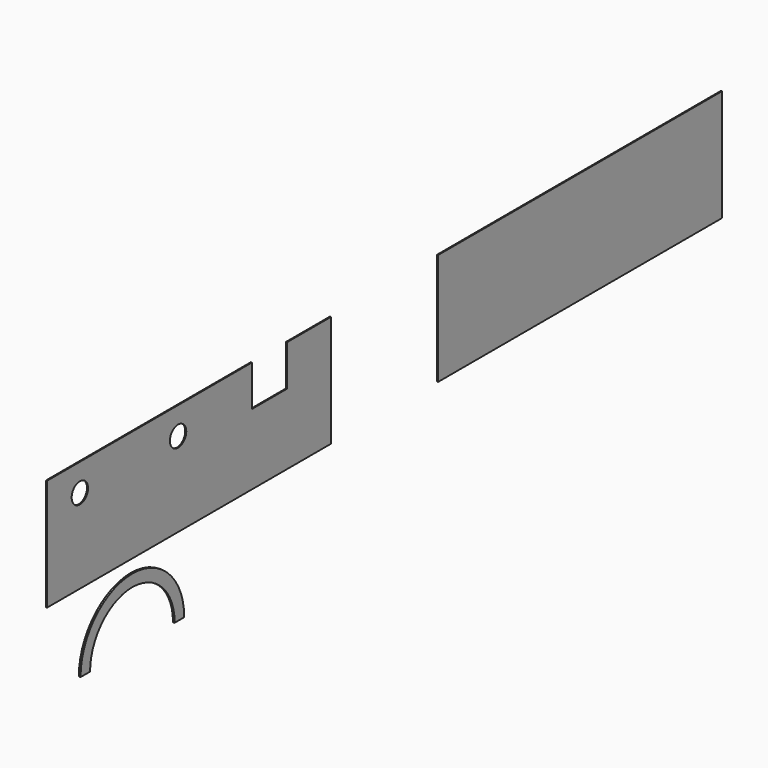
from build123d import *

# Parameters (mm, degrees)
F0_W     = 62
F0_H     = 32.75
F0_R     = 3
F1_DEPTH = 0.3
F0_W_2   = 104
F2_DEPTH = 0.5


# Not quite as in the source:
# - a feature names something its author has since deleted; it is built from what else it names


with BuildPart() as f1:
    # F0 (on Right) → F1 (new body)
    with BuildSketch(Plane.YZ):
        Polygon((-103.3088661638, 20.0492352203), (-61.3088661638, 20.0492352203), (-61.3088661638, 52.7992352203), (-77.3088661638, 52.7992352203), (-77.3088661638, 40.7992352203), (-90.3088661638, 40.7992352203), (-90.3088661638, 52.7992352203), (-103.3088661638, 52.7992352203), align=None)
        with Locations((-134.3088661638, 36.4242352203)):
            Rectangle(F0_W, F0_H)
        with Locations((-153.3088661638, 44.7992352203)):
            Circle(F0_R, mode=Mode.SUBTRACT)
        with Locations((-117.3088661638, 44.7992352203)):
            Circle(F0_R, mode=Mode.SUBTRACT)
    extrude(amount=F1_DEPTH)


with BuildPart() as f1b:
    # F0 (on Right) → F1, piece 2 (new body)
    with BuildSketch(Plane.YZ):
        with Locations((29.9911338362, 36.4242352203)):
            Rectangle(F0_W_2, F0_H)
    extrude(amount=F1_DEPTH)


with BuildPart() as f2:
    # F0 (on Right) → F2 (new body)
    with BuildSketch(Plane.YZ):
        with BuildLine():
            Line((-118.8088661638, -2.7007647797), (-115.3088661638, -2.7007647797))
            ThreePointArc((-115.3088661638, -2.7007647797), (-134.3088661638, 16.2992352203), (-153.3088661638, -2.7007647797))
            Line((-153.3088661638, -2.7007647797), (-149.8088661638, -2.7007647797))
            ThreePointArc((-149.8088661638, -2.7007647797), (-134.3088661638, 12.7992352203), (-118.8088661638, -2.7007647797))
        make_face()
    extrude(amount=F2_DEPTH)


solid = Compound([f1.part, f1b.part, f2.part])
